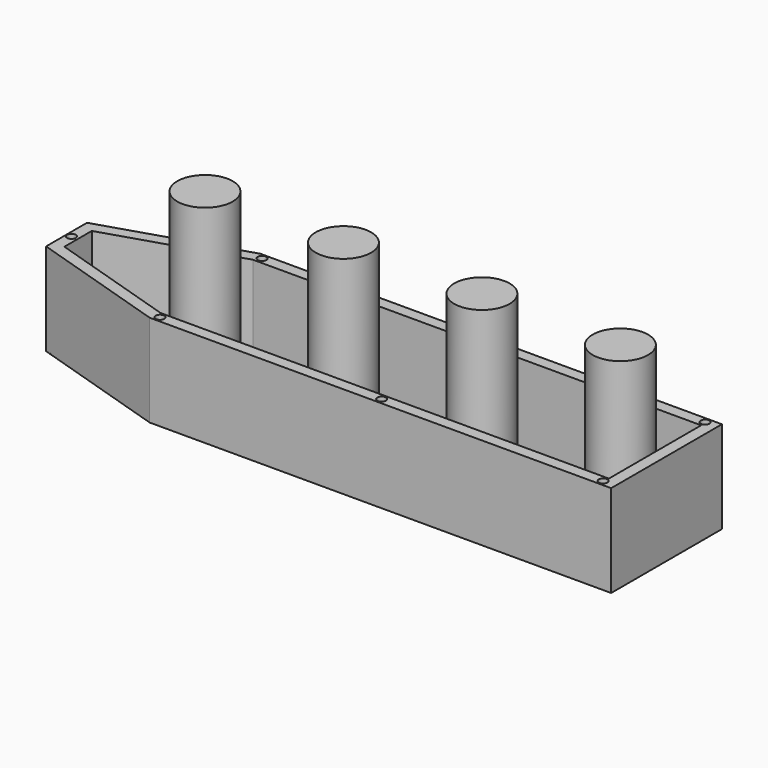
from build123d import *

# Parameters (mm, degrees)
F1_DEPTH      = 25.4
F3_T          = -3.175
F2_R          = 7.62
F4_DEPTH      = 22.86
F4_DEPTH_BACK = 22.225
F5_R          = 1.1967045105
F6_DEPTH      = 7.62
F7_R          = 0.0635
F8_DEPTH      = 12.7


# Not quite as in the source:
# - a feature names something its author has since deleted; it is built from what else it names


with BuildPart() as f1:
    # F0 (on Top) → F1 (new body)
    with BuildSketch(Plane.XY):
        Polygon((-38.1, 7.0371161437), (-38.1, -7.0371161437), (0, -19.05), (127, -19.05), (127, 19.05), (0, 19.05), align=None)
    extrude(amount=F1_DEPTH)

    # F3
    f3_openings = [f1.faces().sort_by_distance(p)[0] for p in [
        (49.931192, 0, 25.4),
    ]]
    offset(amount=F3_T, openings=f3_openings)

    # F2 (on face) → F4 (join, two sides)
    with BuildSketch(Plane.XY.offset(25.4)) as f4_sk:
        Circle(F2_R)
        with Locations((38.1, 0)):
            Circle(F2_R)
        with Locations((76.2, 0)):
            Circle(F2_R)
        with Locations((114.3, 0)):
            Circle(F2_R)
    extrude(amount=F4_DEPTH)
    extrude(f4_sk.sketch, amount=-F4_DEPTH_BACK)

    # F5 (on face) → F6 (cut)
    with BuildSketch(Plane.XY.offset(25.4)):
        with Locations((1.6406770326, 17.5694916397)):
            Circle(F5_R)
        with Locations((62.6006770326, 17.5694916397)):
            Circle(F5_R)
        with Locations((123.5606770326, 17.5694916397)):
            Circle(F5_R)
        with Locations((-36.748547107, 0)):
            Circle(F5_R)
        with Locations((62.6006770326, -17.4930030425)):
            Circle(F5_R)
        with Locations((123.5606770326, -17.4930030425)):
            Circle(F5_R)
        with Locations((1.6406770326, -17.4930030425)):
            Circle(F5_R)
    extrude(amount=-F6_DEPTH, mode=Mode.SUBTRACT)

    # F7 (on face) → F8 (cut)
    with BuildSketch(Plane(origin=(-5.4633155562, -17.3274232219, 0), x_dir=(0.9537169507, -0.3007057995, 0), z_dir=(-0.3007057995, -0.9537169507, 0))):
        with Locations((-32.5760804117, 0.0889)):
            Circle(F7_R)
    extrude(amount=-F8_DEPTH, mode=Mode.SUBTRACT)


solid = f1.part
